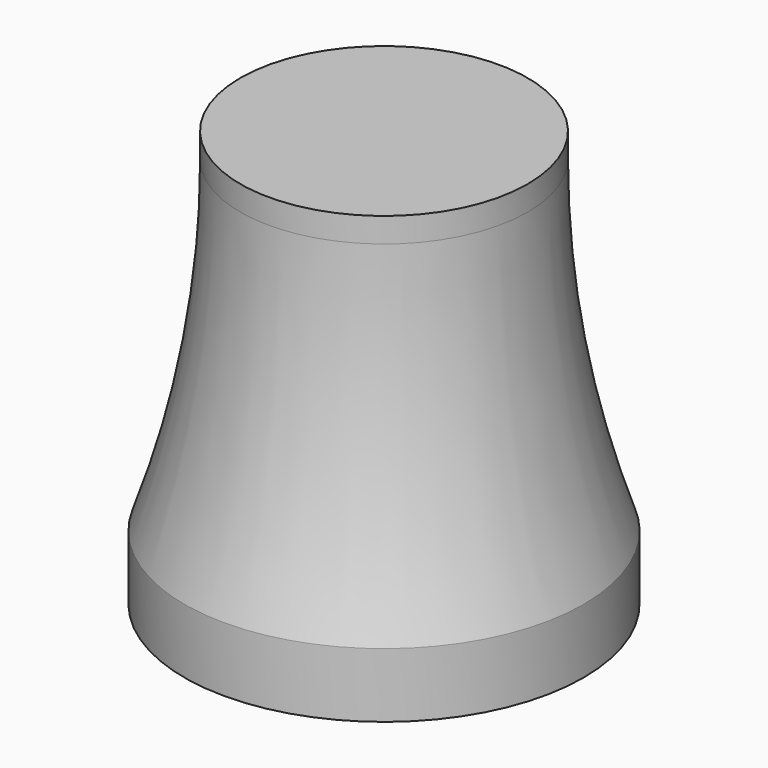
from build123d import *

# Parameters (mm, degrees)
F0_R     = 17.5339973563
F1_DEPTH = 50.8
F2_R     = 24.353495683
F3_DEPTH = 7.874
F5_T     = -7.62


# Not quite as in the source:
# - a fillet or chamfer that OpenCascade refuses, or shapes differently, is made with other operations: its cross-section is extruded or revolved along the edge and cut away or added


with BuildPart() as f1:
    # F0 (on Top) → F1 (new body)
    with BuildSketch(Plane.XY):
        Circle(F0_R)
    extrude(amount=F1_DEPTH)

    # F2 (on Top) → F3 (join)
    with BuildSketch(Plane.XY):
        Circle(F2_R)
    extrude(amount=F3_DEPTH)

    # F4: fillet of radius 120.1892079892 on 1 edges, made by hand

    # F4_s1 → F4_t2 (revolve)
    with BuildSketch(Plane.XZ):
        with BuildLine():
            ThreePointArc((24.353495683, 7.874), (19.2511383183, 27.5394411034), (17.5339973563, 47.7833303391))
            Line((17.5339973563, 47.7833303391), (17.5339973563, 7.874))
            Line((17.5339973563, 7.874), (24.353495683, 7.874))
        make_face()
    revolve(axis=Axis((0, 0, 7.874), (0, 0, -1)))

    # F5
    f5_openings = [f1.faces().sort_by_distance(p)[0] for p in [
        (0, 0, 0),
    ]]
    offset(amount=F5_T, openings=f5_openings)


solid = f1.part
